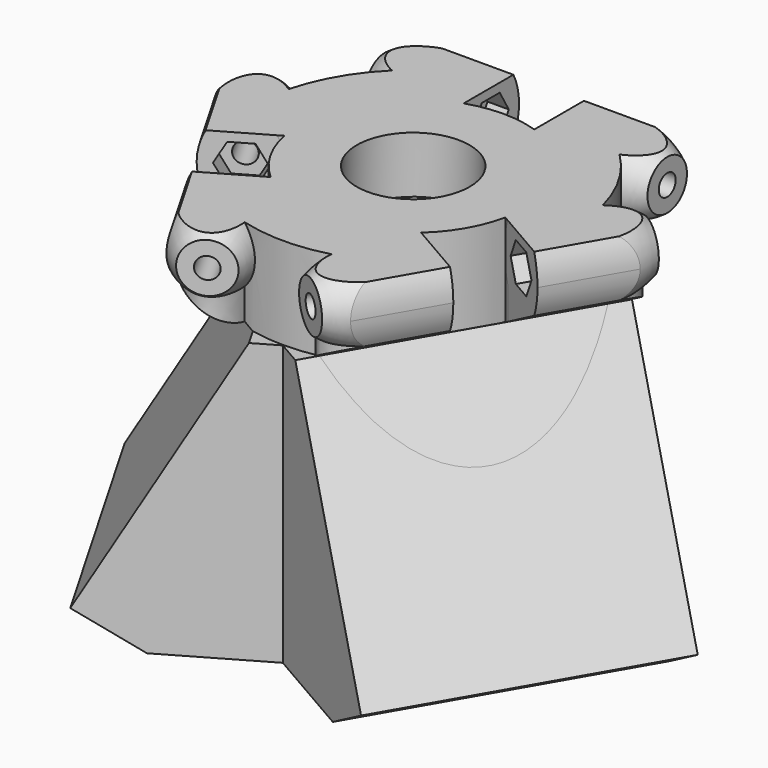
from build123d import *
from build123d import SkipClean  # not in build123d's __all__

# Parameters (mm, degrees)
F1_R      = 3.5
F1_R_2    = 1.5
F2_DEPTH  = 20
F3_DEPTH  = 8
F6_W      = 10
F6_H      = 10
F7_DEPTH  = 12.5
F8_COUNT  = 3
F9_R      = 8
F10_DEPTH = 4
F15_DEPTH = 20
F17_DEPTH = 20
F19_DEPTH = 44.6
F20_DEPTH = 5
F22_DEPTH = 20
F24_DEPTH = 20
F25_R     = 23
F26_DEPTH = 14.6
F27_R     = 11
F28_DEPTH = 44.6
F29_W     = 20
F29_H     = 27
F30_DEPTH = 18.6


with BuildPart() as f2:
    # F1 (on Right) → F2 (new body, symmetric)
    with BuildSketch(Plane.YZ):
        with BuildLine():
            Line((24, 4), (16, 4))
            ThreePointArc((16, 4), (15.2537887488, 2.0615528128), (15, 0))
            ThreePointArc((15, 0), (15.2537887488, -2.0615528128), (16, -4))
            Line((16, -4), (24, -4))
            ThreePointArc((24, -4), (24.7462112512, -2.0615528128), (25, 0))
            ThreePointArc((25, 0), (24.7462112512, 2.0615528128), (24, 4))
        make_face()
        with Locations((20, 0)):
            Circle(F1_R, mode=Mode.SUBTRACT)
        with Locations((20, 0)):
            Circle(F1_R)
        Polygon((16.8245735195, 0), (18.4122867597, 2.75), (21.5877132403, 2.75), (23.1754264805, 0), (21.5877132403, -2.75), (18.4122867597, -2.75), align=None, mode=Mode.SUBTRACT)
        Polygon((21.5877132403, 2.75), (18.4122867597, 2.75), (16.8245735195, 0), (18.4122867597, -2.75), (21.5877132403, -2.75), (23.1754264805, 0), align=None)
        with Locations((20, 0)):
            Circle(F1_R_2, mode=Mode.SUBTRACT)
    extrude(amount=F2_DEPTH, both=True)

    # F1 (on Right) → F3 (cut, symmetric)
    with BuildSketch(Plane.YZ):
        Polygon((21.5877132403, 2.75), (18.4122867597, 2.75), (16.8245735195, 0), (18.4122867597, -2.75), (21.5877132403, -2.75), (23.1754264805, 0), align=None)
        with Locations((20, 0)):
            Circle(F1_R_2, mode=Mode.SUBTRACT)
    extrude(amount=F3_DEPTH, both=True, mode=Mode.SUBTRACT)

    # F4 (on Top) → F5 (revolve, cut)
    with BuildSketch(Plane.XY):
        with BuildLine():
            ThreePointArc((-12, 14), (-16.1907636536, 14.6395563086), (-20, 16.5))
            Line((-20, 16.5), (-20, 14))
            Line((-20, 14), (-12, 14))
        make_face()
        with BuildLine():
            ThreePointArc((20, 16.5), (16.1907636536, 14.6395563086), (12, 14))
            Line((12, 14), (20, 14))
            Line((20, 14), (20, 16.5))
        make_face()
    revolve(axis=Axis((0.2093017101, 20, 0), (1, 0, 0)), mode=Mode.SUBTRACT)

    # F6 (on Top) → F7 (cut, symmetric)
    with BuildSketch(Plane.XY):
        with Locations((0, 20)):
            Rectangle(F6_W, F6_H)
    extrude(amount=F7_DEPTH, both=True, mode=Mode.SUBTRACT)


with BuildPart() as f8_1:
    # F8: instance of F2
    add(f2.part.rotate(Axis((0, 0, 60.3143423796), (0, 0, 1)), 1 * 360 / F8_COUNT), clean=False)


with BuildPart() as f8_2:
    # F8: instance of F2
    add(f2.part.rotate(Axis((0, 0, 60.3143423796), (0, 0, 1)), 2 * 360 / F8_COUNT), clean=False)


with BuildPart() as f2_1:
    add(f2.part, clean=False)

    add(f8_1.part)  # F10 merges F8_1

    add(f8_2.part)  # F10 merges F8_2
    # F9 (on Top) → F10 (join, symmetric)
    with BuildSketch(Plane.XY):
        with BuildLine():
            Line((16.7894191624, -3.9198729811), (22.3011293419, 5.6266890864))
            ThreePointArc((22.3011293419, 5.6266890864), (19.918584287, 11.5), (16.023420359, 16.5))
            Line((16.023420359, 16.5), (5, 16.5))
            Line((5, 16.5), (5, 15.1986841536))
            ThreePointArc((5, 15.1986841536), (12.9614813968, 9.3808315196), (16, 0))
            ThreePointArc((16, 0), (15.9153879201, -1.6432977062), (15.6624465811, -3.2692150579))
            Line((15.6624465811, -3.2692150579), (16.7894191624, -3.9198729811))
        make_face()
        with BuildLine():
            Line((-5, 16.5), (-16.023420359, 16.5))
            ThreePointArc((-16.023420359, 16.5), (-19.918584287, 11.5), (-22.3011293419, 5.6266890864))
            Line((-22.3011293419, 5.6266890864), (-16.7894191624, -3.9198729811))
            Line((-16.7894191624, -3.9198729811), (-15.6624465811, -3.2692150579))
            ThreePointArc((-15.6624465811, -3.2692150579), (-13.8564064606, 8), (-5, 15.1986841536))
            Line((-5, 15.1986841536), (-5, 16.5))
        make_face()
        with BuildLine():
            ThreePointArc((-6.277708983, -22.1266890864), (0, -23), (6.277708983, -22.1266890864))
            Line((6.277708983, -22.1266890864), (11.7894191624, -12.5801270189))
            Line((11.7894191624, -12.5801270189), (10.6624465811, -11.9294690957))
            ThreePointArc((10.6624465811, -11.9294690957), (0, -16), (-10.6624465811, -11.9294690957))
            Line((-10.6624465811, -11.9294690957), (-11.7894191624, -12.5801270189))
            Line((-11.7894191624, -12.5801270189), (-6.277708983, -22.1266890864))
        make_face()
        with BuildLine():
            ThreePointArc((10.6624465811, -11.9294690957), (13.8564064606, -8), (15.6624465811, -3.2692150579))
            ThreePointArc((15.6624465811, -3.2692150579), (15.9153879201, -1.6432977062), (16, 0))
            ThreePointArc((16, 0), (12.9614813968, 9.3808315196), (5, 15.1986841536))
            ThreePointArc((5, 15.1986841536), (0, 16), (-5, 15.1986841536))
            ThreePointArc((-5, 15.1986841536), (-13.8564064606, 8), (-15.6624465811, -3.2692150579))
            ThreePointArc((-15.6624465811, -3.2692150579), (-13.8564064606, -8), (-10.6624465811, -11.9294690957))
            ThreePointArc((-10.6624465811, -11.9294690957), (0, -16), (10.6624465811, -11.9294690957))
        make_face()
        Circle(F9_R, mode=Mode.SUBTRACT)
    extrude(amount=F10_DEPTH, both=True)

    # F14 (on line) → F15 (join, symmetric)
    with BuildSketch(Plane(origin=(0, 0, 0), x_dir=(0.8660254038, 0.5, 0), z_dir=(0.5, -0.8660254038, 0))):
        Polygon((0, -4), (-24, -4), (-15.3397459622, -9), (-35.3397459622, -43.6410161514), (-26.7505339824, -48.6), (0, -48.6), align=None)
    extrude(amount=F15_DEPTH, both=True)

    # F16 (on line) → F17 (join, symmetric)
    with BuildSketch(Plane(origin=(0, 0, 0), x_dir=(-0.8660254038, 0.5, 0), z_dir=(0.5, 0.8660254038, 0))):
        Polygon((0, -48.6), (0, -4), (-24, -4), (-15.3397459622, -9), (-35.3397459622, -43.6410161514), (-26.7505339824, -48.6), align=None)
    extrude(amount=F17_DEPTH, both=True)

    # F18 (on face) → F19 (join)
    with BuildSketch(Plane(origin=(0, 0, -4), x_dir=(1, 0, 0), z_dir=(0, 0, -1))):
        with BuildLine():
            ThreePointArc((-16.1248606678, -16.4008801119), (-15.5710274877, -16.9275840857), (-15, -17.4355957742))
            Line((-15, -17.4355957742), (-15, -14.4337567297))
            Line((-15, -14.4337567297), (-19.8361577865, -11.6415997299))
            ThreePointArc((-19.8361577865, -11.6415997299), (-18.1372930589, -14.1435002915), (-16.1248606678, -16.4008801119))
        make_face()
        with BuildLine():
            Line((15, -14.4337567297), (15, -17.4355957742))
            ThreePointArc((15, -17.4355957742), (15.5710274875, -16.9275840859), (16.1248606673, -16.4008801123))
            ThreePointArc((16.1248606673, -16.4008801123), (18.1372930587, -14.1435002917), (19.8361577865, -11.6415997299))
            Line((19.8361577865, -11.6415997299), (15, -14.4337567297))
        make_face()
        with BuildLine():
            Line((-15, -14.4337567297), (-15, -17.4355957742))
            Line((-15, -17.4355957742), (-5, -17.4355957742))
            Line((-5, -17.4355957742), (-5, -15.1986841536))
            ThreePointArc((-5, -15.1986841536), (0, -16), (5, -15.1986841536))
            Line((5, -15.1986841536), (5, -17.4355957742))
            Line((5, -17.4355957742), (15, -17.4355957742))
            Line((15, -17.4355957742), (15, -14.4337567297))
            Line((15, -14.4337567297), (10, -17.3205080757))
            Line((10, -17.3205080757), (4, -6.9282032303))
            ThreePointArc((4, -6.9282032303), (0, -8), (-4, -6.9282032303))
            Line((-4, -6.9282032303), (-10, -17.3205080757))
            Line((-10, -17.3205080757), (-15, -14.4337567297))
        make_face()
        with BuildLine():
            Line((-15, -3.1848524231), (-15, -14.4337567297))
            Line((-15, -14.4337567297), (-10, -17.3205080757))
            Line((-10, -17.3205080757), (-4, -6.9282032303))
            ThreePointArc((-4, -6.9282032303), (0, -8), (4, -6.9282032303))
            Line((4, -6.9282032303), (10, -17.3205080757))
            Line((10, -17.3205080757), (15, -14.4337567297))
            Line((15, -14.4337567297), (15, -3.1848524231))
            Line((15, -3.1848524231), (-15, -3.1848524231))
        make_face()
        with BuildLine():
            Line((-19.8361577865, -11.6415997299), (-15, -14.4337567297))
            Line((-15, -14.4337567297), (-15, -3.1848524231))
            Line((-15, -3.1848524231), (15, -3.1848524231))
            Line((15, -3.1848524231), (15, -14.4337567297))
            Line((15, -14.4337567297), (19.8361577865, -11.6415997299))
            ThreePointArc((19.8361577865, -11.6415997299), (22.1949502037, -6.0319304916), (23, 0))
            ThreePointArc((23, 0), (-6.0319304916, 22.1949502037), (-19.8361577865, -11.6415997299))
        make_face()
        with BuildLine():
            Line((-5, -15.1986841536), (-5, -17.4355957742))
            Line((-5, -17.4355957742), (5, -17.4355957742))
            Line((5, -17.4355957742), (5, -15.1986841536))
            ThreePointArc((5, -15.1986841536), (0, -16), (-5, -15.1986841536))
        make_face()
    extrude(amount=F19_DEPTH)

    # F20 (cut): faces of the model
    f20_faces = [f2_1.faces().sort_by_distance(p)[0] for p in [
        (-25.232335449, 7.1039673105, -4),
        (-5.5294682322, -25.9696854669, -4),
        (16.6921842183, -9.6372370518, -4),
        (20.2627727519, -11.6987173028, -4),
        (25.2323372994, 7.1039664149, -4),
        (0, -1.0185916358, -4),
        (25.2323372994, 7.1039664149, -4),
        (0, -1.0185916358, -4),
        (16.6921842183, -9.6372370518, -4),
        (20.2627727519, -11.6987173028, -4),
        (-20.2627727519, -11.6987173028, -4),
        (-16.6921842183, -9.6372370518, -4),
    ]]
    with SkipClean():  # cleaning this boolean's faces spoils the solid; the shape is the same uncleaned
        extrude(f20_faces, amount=-F20_DEPTH, mode=Mode.SUBTRACT)

    # F21 (on line) → F22 (cut, symmetric)
    with BuildSketch(Plane(origin=(0, 0, 0), x_dir=(0.8660254038, 0.5, 0), z_dir=(0.5, -0.8660254038, 0))):
        Polygon((-15.3397459622, -9), (-24, -4), (-24.2418040845, -24.4188169598), align=None)
    with SkipClean():  # cleaning this boolean's faces spoils the solid; the shape is the same uncleaned
        extrude(amount=F22_DEPTH, both=True, mode=Mode.SUBTRACT)

    # F23 (on line) → F24 (cut, symmetric)
    with BuildSketch(Plane(origin=(0, 0, 0), x_dir=(-0.8660254038, 0.5, 0), z_dir=(0.5, 0.8660254038, 0))):
        Polygon((-25.5929308491, -26.7590371636), (-15.3397459622, -9), (-24, -4), align=None)
    extrude(amount=F24_DEPTH, both=True, mode=Mode.SUBTRACT)

    # F25 (on face) → F26 (join)
    with BuildSketch(Plane(origin=(0, 0, -48.6), x_dir=(1, 0, 0), z_dir=(0, 0, -1))):
        Circle(F25_R)
    extrude(amount=-F26_DEPTH)

    # F27 (on face) → F28 (cut)
    with BuildSketch(Plane(origin=(0, 0, -48.6), x_dir=(1, 0, 0), z_dir=(0, 0, -1))):
        Circle(F27_R)
    extrude(amount=-F28_DEPTH, mode=Mode.SUBTRACT)

    # F29 (on face) → F30 (cut)
    with BuildSketch(Plane(origin=(0, 0, -48.6), x_dir=(1, 0, 0), z_dir=(0, 0, -1))):
        with Locations((0, -3.5)):
            Rectangle(F29_W, F29_H)
    extrude(amount=-F30_DEPTH, mode=Mode.SUBTRACT)


solid = f2_1.part
